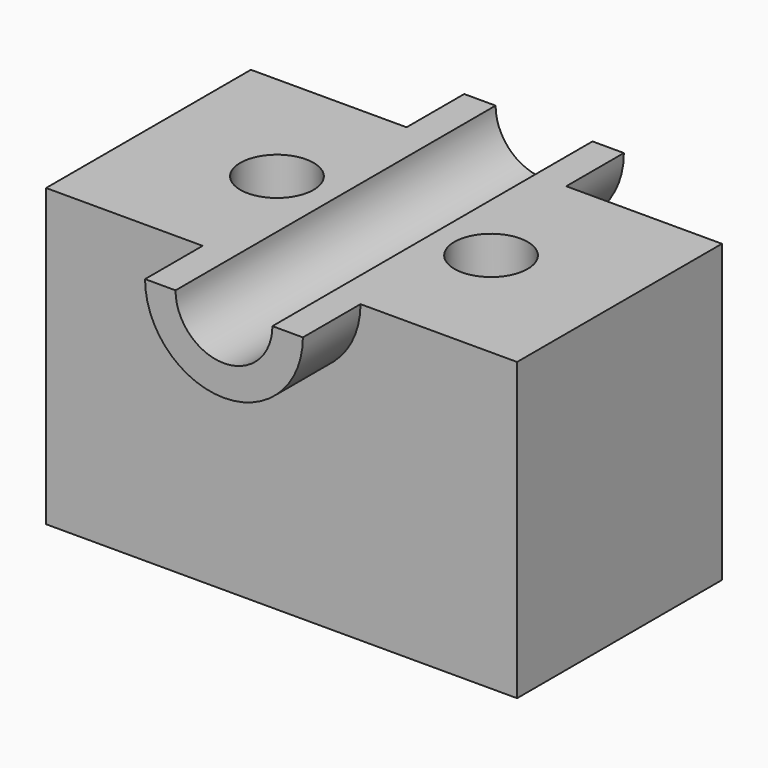
from build123d import *

# Parameters (mm, degrees)
F0_W       = 166.1031842232
F0_H       = 90.2919918299
F1_DEPTH   = 104.394
F1_FACE1_W = 166.1031842232
F1_FACE1_H = 104.394
F3_DEPTH   = 25.4
F5_DEPTH   = 306.324
F7_DEPTH   = 25.4
F8_R       = 12.9217505793
F9_DEPTH   = 104.395


# Not quite as in the source:
# - a pattern or mirror of a feature is missing from the dataset's text; its kind, count and spacing are read off the source's solid


with BuildPart() as f1:
    # F0 (on Top) → F1 (new body)
    with BuildSketch(Plane.XY):
        Rectangle(F0_W, F0_H)
    extrude(amount=F1_DEPTH)

    # F2 (on face) + F1_face1 (on face) → F3 (join)
    with BuildSketch(Plane(origin=(0, 45.1459959149, 0), x_dir=(-1, 0, 0), z_dir=(0, 1, 0))):
        with BuildLine():
            Line((28.1535676802, 104.394), (17.0834749636, 104.394))
            ThreePointArc((17.0834749636, 104.394), (0, 87.3105250364), (-17.0834749636, 104.394))
            Line((-17.0834749636, 104.394), (-28.1535676802, 104.394))
            ThreePointArc((-28.1535676802, 104.394), (0, 76.2404323198), (28.1535676802, 104.394))
        make_face()
    with BuildSketch(Plane(origin=(0, -45.1459959149, 52.197), x_dir=(1, 0, 0), z_dir=(0, -1, 0))):
        Rectangle(F1_FACE1_W, F1_FACE1_H)
    extrude(amount=F3_DEPTH, dir=(0, 1, 0))

    # F4 (on face) → F5 (cut)
    with BuildSketch(Plane(origin=(0, 45.1459959149, 0), x_dir=(-1, 0, 0), z_dir=(0, 1, 0))):
        with BuildLine():
            Line((17.0834749636, 104.394), (-17.0834749636, 104.394))
            ThreePointArc((-17.0834749636, 104.394), (0, 87.3105250364), (17.0834749636, 104.394))
        make_face()
    extrude(amount=-F5_DEPTH, mode=Mode.SUBTRACT)

    # F6 (on face) → F7 (join)
    with BuildSketch(Plane.XZ.offset(45.1459959149)):
        with BuildLine():
            ThreePointArc((-27.8307711085, 104.394), (0, 76.5632288915), (27.8307711085, 104.394))
            Line((27.8307711085, 104.394), (17.0834749636, 104.394))
            ThreePointArc((17.0834749636, 104.394), (0, 87.3105250364), (-17.0834749636, 104.394))
            Line((-17.0834749636, 104.394), (-27.8307711085, 104.394))
        make_face()
    extrude(amount=F7_DEPTH)

    # F8 (on face) → F9 (cut, through all)
    with BuildSketch(Plane.XY.offset(104.394)):
        with Locations((37.7448610961, 0)):
            Circle(F8_R)
    f9 = extrude(amount=-F9_DEPTH, mode=Mode.SUBTRACT)

    # F9_copies: F9 across plane
    add(f9.mirror(Plane(origin=(0, 0, 0), x_dir=(0, 0, -1), z_dir=(-1, 0, 0))), mode=Mode.SUBTRACT)


solid = f1.part
